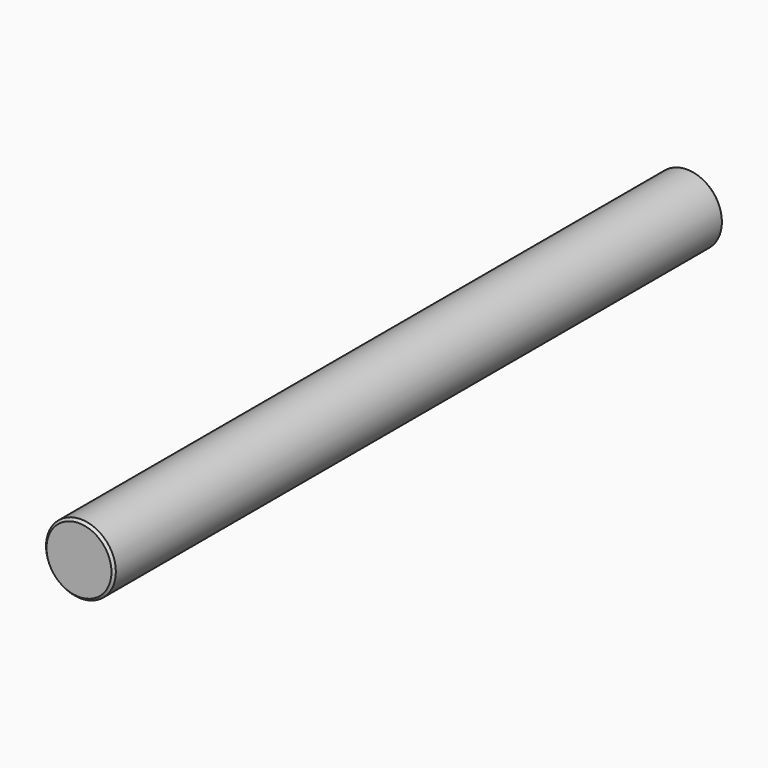
from build123d import *

# Parameters (mm, degrees)
F0_R     = 136.525
F0_R_2   = 127
F1_DEPTH = 2981.325
F2_SIZE  = 9.52499


# Not quite as in the source:
# - a fillet or chamfer is up to 0.001 mm smaller than in the source, because OpenCascade refuses the exact size


with BuildPart() as f1:
    # F0 (on Front) → F1 (new body)
    with BuildSketch(Plane.XZ):
        Circle(F0_R)
        Circle(F0_R_2, mode=Mode.SUBTRACT)
    extrude(amount=F1_DEPTH)

    # F2 (size 9.525 in the source; OpenCascade refuses exactly that, so slightly less here)
    f2_edges = [f1.edges().sort_by_distance(p)[0] for p in [
        (-136.525, 0, 0),
        (-136.525, -2981.325, 0),
    ]]
    chamfer(f2_edges, length=F2_SIZE)


solid = f1.part
